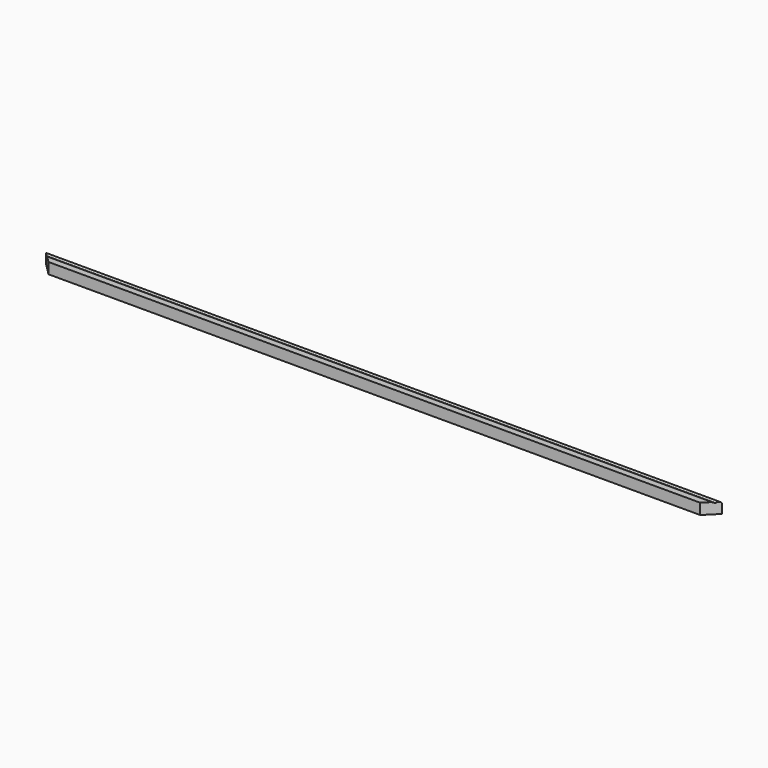
from build123d import *

# Parameters (mm, degrees)
F1_DEPTH = 889
F2_SIZE  = 31.74999


# Not quite as in the source:
# - a fillet or chamfer is up to 0.001 mm smaller than in the source, because OpenCascade refuses the exact size


with BuildPart() as f1:
    # F0 (on Right) → F1 (new body, symmetric)
    with BuildSketch(Plane.YZ):
        with BuildLine():
            Line((-15.875, -14.2875), (15.875, -14.2875))
            Line((15.875, -14.2875), (15.875, 9.525))
            ThreePointArc((15.875, 9.525), (12.4385421004, 14.0991686237), (7.08843051, 12.07220847))
            ThreePointArc((7.08843051, 12.07220847), (5.9853917743, 11.4055483551), (4.789455264, 11.886033552))
            ThreePointArc((4.789455264, 11.886033552), (2.3755826554, 13.6595328458), (-0.5531949, 14.2875))
            Line((-0.5531949, 14.2875), (-15.875, 14.2875))
            Line((-15.875, 14.2875), (-15.875, -14.2875))
        make_face()
    extrude(amount=F1_DEPTH, both=True)

    # F2 (size 31.75 in the source; OpenCascade refuses exactly that, so slightly less here)
    f2_edges = [f1.edges().sort_by_distance(p)[0] for p in [
        (-889, -15.875, 0),
        (889, -15.875, 0),
    ]]
    chamfer(f2_edges, length=F2_SIZE)


solid = f1.part
